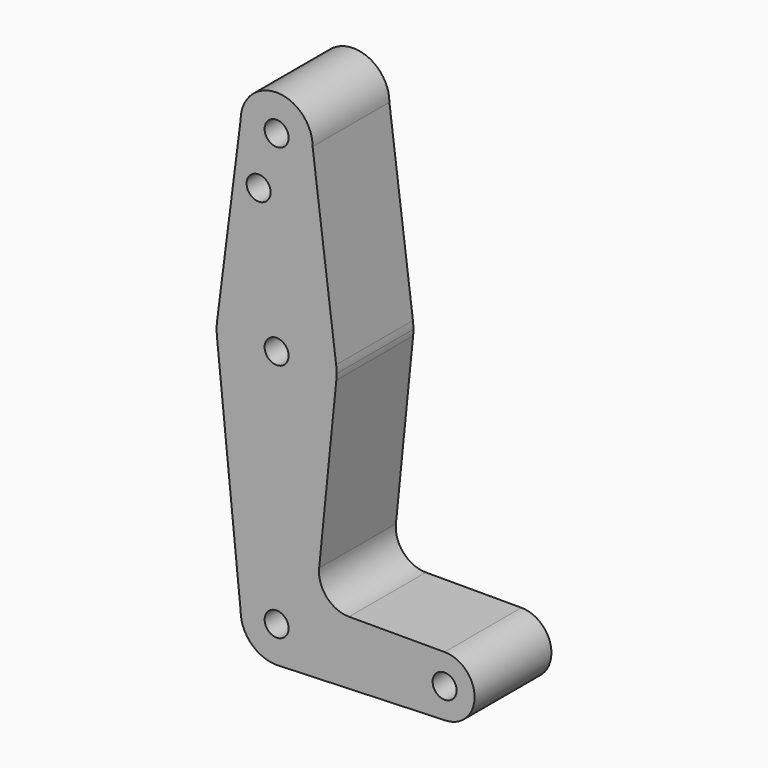
from build123d import *

# Parameters (mm, degrees)
F0_R     = 3.175
F1_DEPTH = 25.4


# Not quite as in the source:
# - ends of sketch curves that miss each other by under 0.0002 mm in the source are joined


with BuildPart() as f1:
    # F0 (on Front) → F1 (new body)
    with BuildSketch(Plane.XZ):
        with BuildLine():
            ThreePointArc((9.525, 114.3), (0, 123.825), (-9.525, 114.3))
            ThreePointArc((-9.525, 114.3), (0, 104.775), (9.525, 114.3))
        make_face()
        with Locations((0, 114.3)):
            Circle(F0_R, mode=Mode.SUBTRACT)
        with BuildLine():
            Line((-9.525, 114.3), (-15.7474569047, 65.5082893304))
            ThreePointArc((-15.7474569047, 65.5082893304), (0, 79.375), (15.7474569047, 65.5082893304))
            Line((15.7474569047, 65.5082893304), (9.525, 114.3))
            ThreePointArc((9.525, 114.3), (0, 104.775), (-9.525, 114.3))
        make_face()
        with Locations((-4.7625, 100.0252)):
            Circle(F0_R, mode=Mode.SUBTRACT)
        with BuildLine():
            ThreePointArc((-9.525, 0), (0, 9.525), (9.525, 0))
            ThreePointArc((9.525, 0), (6.9705567315, -6.4912990883), (0.6773435479, -9.500885786))
            Line((0.6773435479, -9.500885786), (44.7324052746, -7.9324746146))
            ThreePointArc((44.7324052746, -7.9324746146), (36.5137564458, -0.1412249921), (44.45, 7.9375))
            Line((44.45, 7.9375), (19.160010759, 7.9375))
            ThreePointArc((19.160010759, 7.9375), (13.2639846378, 10.5545437096), (11.2496616365, 16.68272))
            Line((11.2496616365, 16.68272), (15.7954255641, 61.9125))
            ThreePointArc((15.7954255641, 61.9125), (15.8550939106, 62.7052534459), (15.875, 63.5))
            ThreePointArc((15.875, 63.5), (15.8430821396, 64.5061676396), (15.7474569047, 65.5082893304))
            ThreePointArc((15.7474569047, 65.5082893304), (0, 79.375), (-15.7474569047, 65.5082893304))
            ThreePointArc((-15.7474569047, 65.5082893304), (-15.8735876139, 63.7117575563), (-15.795425611, 61.9125004674))
            Line((-15.795425611, 61.9125004674), (-9.525, 0))
        make_face()
        with Locations((0, 63.5)):
            Circle(F0_R, mode=Mode.SUBTRACT)
        with BuildLine():
            ThreePointArc((0.6773435479, -9.500885786), (6.9705567315, -6.4912990883), (9.525, 0))
            ThreePointArc((9.525, 0), (0, 9.525), (-9.525, 0))
            ThreePointArc((-9.525, 0), (-6.7351920908, -6.7351920908), (0, -9.525))
            Line((0, -9.525), (0.6773435479, -9.500885786))
        make_face()
        Circle(F0_R, mode=Mode.SUBTRACT)
        with BuildLine():
            ThreePointArc((44.45, 7.9375), (36.5137564458, -0.1412249921), (44.7324052746, -7.9324746146))
            ThreePointArc((44.7324052746, -7.9324746146), (50.1616327839, -5.5119104847), (52.3875, 0))
            ThreePointArc((52.3875, 0), (50.0626600757, 5.6126600757), (44.45, 7.9375))
        make_face()
        with Locations((44.45, 0)):
            Circle(F0_R, mode=Mode.SUBTRACT)
    extrude(amount=F1_DEPTH)


solid = f1.part
